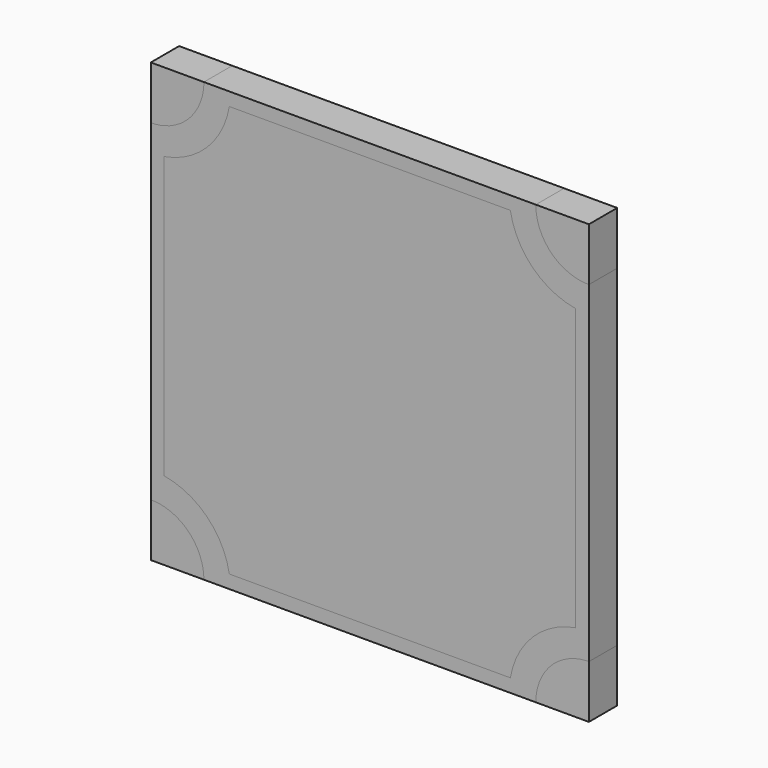
from build123d import *

# Parameters (mm, degrees)
F2_DEPTH = 6.35
F3_DEPTH = 6.35
F1_W     = 2.38125
F1_H     = 2.38125
F4_DEPTH = 6.35


with BuildPart() as f2:
    # F1 (on face) → F2 (new body)
    with BuildSketch(Plane.XZ):
        with BuildLine():
            Line((-76.2, 64.4935850165), (-76.2, 14.0876649835))
            ThreePointArc((-76.2, 14.0876649835), (-68.4784618638, 10.1027881362), (-64.4935850165, 2.38125))
            Line((-64.4935850165, 2.38125), (-14.0876649835, 2.38125))
            ThreePointArc((-14.0876649835, 2.38125), (-10.1027881362, 10.1027881362), (-2.38125, 14.0876649835))
            Line((-2.38125, 14.0876649835), (-2.38125, 64.4935850165))
            ThreePointArc((-2.38125, 64.4935850165), (-10.1027881362, 68.4784618638), (-14.0876649835, 76.2))
            Line((-14.0876649835, 76.2), (-64.4935850165, 76.2))
            ThreePointArc((-64.4935850165, 76.2), (-68.4784618638, 68.4784618638), (-76.2, 64.4935850165))
        make_face()
    extrude(amount=F2_DEPTH)


with BuildPart() as f3:
    # F1 (on face) → F3 (new body)
    with BuildSketch(Plane.XZ):
        with BuildLine():
            Line((-76.2, 76.2), (-76.2, 69.3587084068))
            ThreePointArc((-76.2, 69.3587084068), (-71.8460579092, 71.8460579092), (-69.3587084068, 76.2))
            Line((-69.3587084068, 76.2), (-76.2, 76.2))
        make_face()
        with BuildLine():
            Line((-78.58125, 78.58125), (-78.58125, 69.05625))
            ThreePointArc((-78.58125, 69.05625), (-77.3810591141, 69.1321671431), (-76.2, 69.3587084068))
            Line((-76.2, 69.3587084068), (-76.2, 76.2))
            Line((-76.2, 76.2), (-69.3587084068, 76.2))
            ThreePointArc((-69.3587084068, 76.2), (-69.1321671431, 77.3810591141), (-69.05625, 78.58125))
            Line((-69.05625, 78.58125), (-78.58125, 78.58125))
        make_face()
    extrude(amount=F3_DEPTH)


with BuildPart() as f3b:
    # F1 (on face) → F3, piece 2 (new body)
    with BuildSketch(Plane.XZ):
        with BuildLine():
            Line((-2.38125, 76.2), (-9.2225415932, 76.2))
            ThreePointArc((-9.2225415932, 76.2), (-6.7351920908, 71.8460579092), (-2.38125, 69.3587084068))
            Line((-2.38125, 69.3587084068), (-2.38125, 76.2))
        make_face()
        with BuildLine():
            ThreePointArc((-2.38125, 69.3587084068), (-1.2001908859, 69.1321671431), (0, 69.05625))
            Line((0, 69.05625), (0, 76.2))
            Line((0, 76.2), (-2.38125, 76.2))
            Line((-2.38125, 76.2), (-2.38125, 69.3587084068))
        make_face()
        with BuildLine():
            Line((0, 78.58125), (-9.525, 78.58125))
            ThreePointArc((-9.525, 78.58125), (-9.4490828569, 77.3810591141), (-9.2225415932, 76.2))
            Line((-9.2225415932, 76.2), (-2.38125, 76.2))
            Line((-2.38125, 76.2), (0, 76.2))
            Line((0, 76.2), (0, 78.58125))
        make_face()
    extrude(amount=F3_DEPTH)


with BuildPart() as f3c:
    # F1 (on face) → F3, piece 3 (new body)
    with BuildSketch(Plane.XZ):
        with BuildLine():
            ThreePointArc((-9.2225415932, 2.38125), (-9.4490828569, 1.2001908859), (-9.525, 0))
            Line((-9.525, 0), (-2.38125, 0))
            Line((-2.38125, 0), (-2.38125, 2.38125))
            Line((-2.38125, 2.38125), (-9.2225415932, 2.38125))
        make_face()
        with BuildLine():
            ThreePointArc((-2.38125, 9.2225415932), (-6.7351920908, 6.7351920908), (-9.2225415932, 2.38125))
            Line((-9.2225415932, 2.38125), (-2.38125, 2.38125))
            Line((-2.38125, 2.38125), (-2.38125, 9.2225415932))
        make_face()
        with Locations((-1.190625, 1.190625)):
            Rectangle(F1_W, F1_H)
        with BuildLine():
            Line((-2.38125, 2.38125), (0, 2.38125))
            Line((0, 2.38125), (0, 9.525))
            ThreePointArc((0, 9.525), (-1.2001908859, 9.4490828569), (-2.38125, 9.2225415932))
            Line((-2.38125, 9.2225415932), (-2.38125, 2.38125))
        make_face()
    extrude(amount=F3_DEPTH)


with BuildPart() as f3d:
    # F1 (on face) → F3, piece 4 (new body)
    with BuildSketch(Plane.XZ):
        with BuildLine():
            ThreePointArc((-69.3587084068, 2.38125), (-71.8460579092, 6.7351920908), (-76.2, 9.2225415932))
            Line((-76.2, 9.2225415932), (-76.2, 2.38125))
            Line((-76.2, 2.38125), (-69.3587084068, 2.38125))
        make_face()
        with BuildLine():
            Line((-76.2, 2.38125), (-76.2, 0))
            Line((-76.2, 0), (-69.05625, 0))
            ThreePointArc((-69.05625, 0), (-69.1321671431, 1.2001908859), (-69.3587084068, 2.38125))
            Line((-69.3587084068, 2.38125), (-76.2, 2.38125))
        make_face()
        with BuildLine():
            Line((-78.58125, 9.525), (-78.58125, 0))
            Line((-78.58125, 0), (-76.2, 0))
            Line((-76.2, 0), (-76.2, 2.38125))
            Line((-76.2, 2.38125), (-76.2, 9.2225415932))
            ThreePointArc((-76.2, 9.2225415932), (-77.3810591141, 9.4490828569), (-78.58125, 9.525))
        make_face()
    extrude(amount=F3_DEPTH)


with BuildPart() as f4:
    # F1 (on face) → F4 (new body)
    with BuildSketch(Plane.XZ):
        with BuildLine():
            ThreePointArc((-64.4935850165, 76.2), (-64.3437964057, 77.3864398063), (-64.29375, 78.58125))
            Line((-64.29375, 78.58125), (-69.05625, 78.58125))
            ThreePointArc((-69.05625, 78.58125), (-69.1321671431, 77.3810591141), (-69.3587084068, 76.2))
            Line((-69.3587084068, 76.2), (-64.4935850165, 76.2))
        make_face()
        with BuildLine():
            Line((-76.2, 69.3587084068), (-76.2, 64.4935850165))
            ThreePointArc((-76.2, 64.4935850165), (-68.4784618638, 68.4784618638), (-64.4935850165, 76.2))
            Line((-64.4935850165, 76.2), (-69.3587084068, 76.2))
            ThreePointArc((-69.3587084068, 76.2), (-71.8460579092, 71.8460579092), (-76.2, 69.3587084068))
        make_face()
        with BuildLine():
            Line((-78.58125, 69.05625), (-78.58125, 64.29375))
            ThreePointArc((-78.58125, 64.29375), (-77.3864398063, 64.3437964057), (-76.2, 64.4935850165))
            Line((-76.2, 64.4935850165), (-76.2, 69.3587084068))
            ThreePointArc((-76.2, 69.3587084068), (-77.3810591141, 69.1321671431), (-78.58125, 69.05625))
        make_face()
        with BuildLine():
            Line((-78.58125, 64.29375), (-78.58125, 14.2875))
            ThreePointArc((-78.58125, 14.2875), (-77.3864398063, 14.2374535943), (-76.2, 14.0876649835))
            Line((-76.2, 14.0876649835), (-76.2, 64.4935850165))
            ThreePointArc((-76.2, 64.4935850165), (-77.3864398063, 64.3437964057), (-78.58125, 64.29375))
        make_face()
        with BuildLine():
            ThreePointArc((-76.2, 14.0876649835), (-77.3864398063, 14.2374535943), (-78.58125, 14.2875))
            Line((-78.58125, 14.2875), (-78.58125, 9.525))
            ThreePointArc((-78.58125, 9.525), (-77.3810591141, 9.4490828569), (-76.2, 9.2225415932))
            Line((-76.2, 9.2225415932), (-76.2, 14.0876649835))
        make_face()
        with BuildLine():
            ThreePointArc((-64.4935850165, 2.38125), (-68.4784618638, 10.1027881362), (-76.2, 14.0876649835))
            Line((-76.2, 14.0876649835), (-76.2, 9.2225415932))
            ThreePointArc((-76.2, 9.2225415932), (-71.8460579092, 6.7351920908), (-69.3587084068, 2.38125))
            Line((-69.3587084068, 2.38125), (-64.4935850165, 2.38125))
        make_face()
        with BuildLine():
            Line((-69.05625, 0), (-64.29375, 0))
            ThreePointArc((-64.29375, 0), (-64.3437964057, 1.1948101937), (-64.4935850165, 2.38125))
            Line((-64.4935850165, 2.38125), (-69.3587084068, 2.38125))
            ThreePointArc((-69.3587084068, 2.38125), (-69.1321671431, 1.2001908859), (-69.05625, 0))
        make_face()
        with BuildLine():
            Line((-64.29375, 0), (-14.2875, 0))
            ThreePointArc((-14.2875, 0), (-14.2374535943, 1.1948101937), (-14.0876649835, 2.38125))
            Line((-14.0876649835, 2.38125), (-64.4935850165, 2.38125))
            ThreePointArc((-64.4935850165, 2.38125), (-64.3437964057, 1.1948101937), (-64.29375, 0))
        make_face()
        with BuildLine():
            ThreePointArc((-2.38125, 14.0876649835), (-10.1027881362, 10.1027881362), (-14.0876649835, 2.38125))
            Line((-14.0876649835, 2.38125), (-9.2225415932, 2.38125))
            ThreePointArc((-9.2225415932, 2.38125), (-6.7351920908, 6.7351920908), (-2.38125, 9.2225415932))
            Line((-2.38125, 9.2225415932), (-2.38125, 14.0876649835))
        make_face()
        with BuildLine():
            ThreePointArc((-14.0876649835, 2.38125), (-14.2374535943, 1.1948101937), (-14.2875, 0))
            Line((-14.2875, 0), (-9.525, 0))
            ThreePointArc((-9.525, 0), (-9.4490828569, 1.2001908859), (-9.2225415932, 2.38125))
            Line((-9.2225415932, 2.38125), (-14.0876649835, 2.38125))
        make_face()
        with BuildLine():
            ThreePointArc((-2.38125, 14.0876649835), (-1.1948101937, 14.2374535943), (0, 14.2875))
            Line((0, 14.2875), (0, 64.29375))
            ThreePointArc((0, 64.29375), (-1.1948101937, 64.3437964057), (-2.38125, 64.4935850165))
            Line((-2.38125, 64.4935850165), (-2.38125, 14.0876649835))
        make_face()
        with BuildLine():
            Line((-9.2225415932, 76.2), (-14.0876649835, 76.2))
            ThreePointArc((-14.0876649835, 76.2), (-10.1027881362, 68.4784618638), (-2.38125, 64.4935850165))
            Line((-2.38125, 64.4935850165), (-2.38125, 69.3587084068))
            ThreePointArc((-2.38125, 69.3587084068), (-6.7351920908, 71.8460579092), (-9.2225415932, 76.2))
        make_face()
        with BuildLine():
            ThreePointArc((-2.38125, 64.4935850165), (-1.1948101937, 64.3437964057), (0, 64.29375))
            Line((0, 64.29375), (0, 69.05625))
            ThreePointArc((0, 69.05625), (-1.2001908859, 69.1321671431), (-2.38125, 69.3587084068))
            Line((-2.38125, 69.3587084068), (-2.38125, 64.4935850165))
        make_face()
        with BuildLine():
            Line((-9.525, 78.58125), (-14.2875, 78.58125))
            ThreePointArc((-14.2875, 78.58125), (-14.2374535943, 77.3864398063), (-14.0876649835, 76.2))
            Line((-14.0876649835, 76.2), (-9.2225415932, 76.2))
            ThreePointArc((-9.2225415932, 76.2), (-9.4490828569, 77.3810591141), (-9.525, 78.58125))
        make_face()
        with BuildLine():
            Line((-14.2875, 78.58125), (-64.29375, 78.58125))
            ThreePointArc((-64.29375, 78.58125), (-64.3437964057, 77.3864398063), (-64.4935850165, 76.2))
            Line((-64.4935850165, 76.2), (-14.0876649835, 76.2))
            ThreePointArc((-14.0876649835, 76.2), (-14.2374535943, 77.3864398063), (-14.2875, 78.58125))
        make_face()
        with BuildLine():
            Line((0, 9.525), (0, 14.2875))
            ThreePointArc((0, 14.2875), (-1.1948101937, 14.2374535943), (-2.38125, 14.0876649835))
            Line((-2.38125, 14.0876649835), (-2.38125, 9.2225415932))
            ThreePointArc((-2.38125, 9.2225415932), (-1.2001908859, 9.4490828569), (0, 9.525))
        make_face()
    extrude(amount=F4_DEPTH)


solid = Compound([f2.part, f3.part, f3b.part, f3c.part, f3d.part, f4.part])
